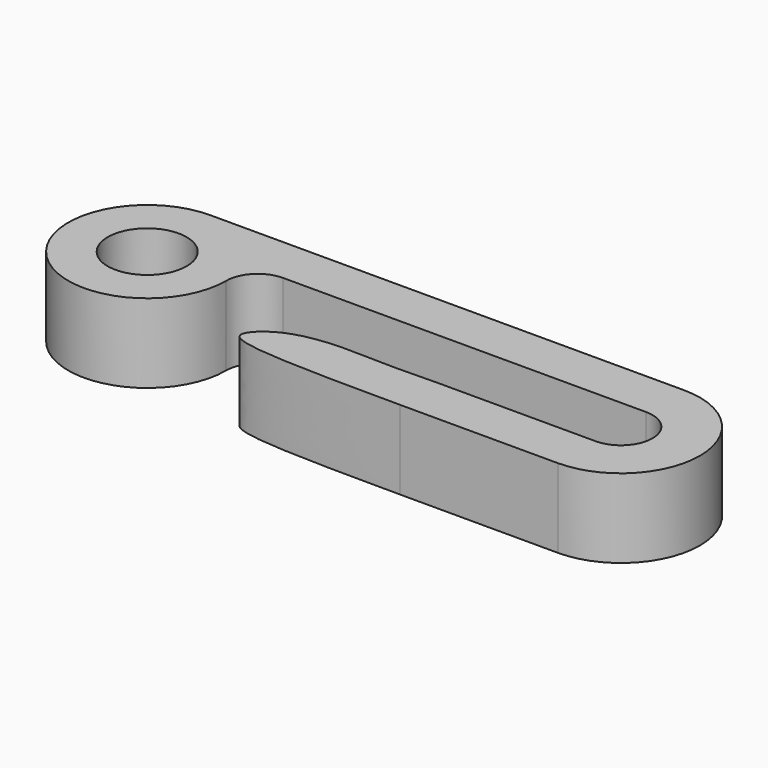
from build123d import *

# Parameters (mm, degrees)
F0_R     = 5
F1_DEPTH = 10


# Not quite as in the source:
# - ends of sketch curves that miss each other by under 0.0002 mm in the source are joined


with BuildPart() as f1:
    # F0 (on Top) → F1 (new body)
    with BuildSketch(Plane.XY):
        with BuildLine():
            ThreePointArc((-30.0000003377, 9.9974011055), (-30.0000000844, 9.9987005527), (-30, 10))
            ThreePointArc((-30, 10), (-32.9289321881, 17.0710678119), (-40, 20))
            ThreePointArc((-40, 20), (-47.0719866001, 2.9298510958), (-30.0000003377, 9.9974011055))
        make_face()
        with Locations((-40, 10)):
            Circle(F0_R, mode=Mode.SUBTRACT)
        with BuildLine():
            ThreePointArc((-40, 20), (-32.9289321881, 17.0710678119), (-30, 10))
            ThreePointArc((-30, 10), (-28.8260746289, 12.8286475986), (-25.9963610747, 14))
            Line((-25.9963610747, 14), (20, 14))
            ThreePointArc((20, 14), (24, 10), (20, 6))
            Line((20, 6), (0, 6))
            add(Edge.make_bspline(
                [(0, 0), (-18.0512891521, 0), (-23.9813730686, 0.6377710425), (-18.8085221866, 5.3625723562), (-11.4536762775, 6.3679885575), (-6.8766033776, 5.7466003341), (0, 6)],
                knots=[0, 0, 0, 0, 0.3683888151, 0.5191562868, 0.7199539542, 1, 1, 1, 1], degree=3))
            Line((0, 0), (20, 0))
            ThreePointArc((20, 0), (30, 10), (20, 20))
            Line((20, 20), (-40, 20))
        make_face()
    extrude(amount=F1_DEPTH)


solid = f1.part
